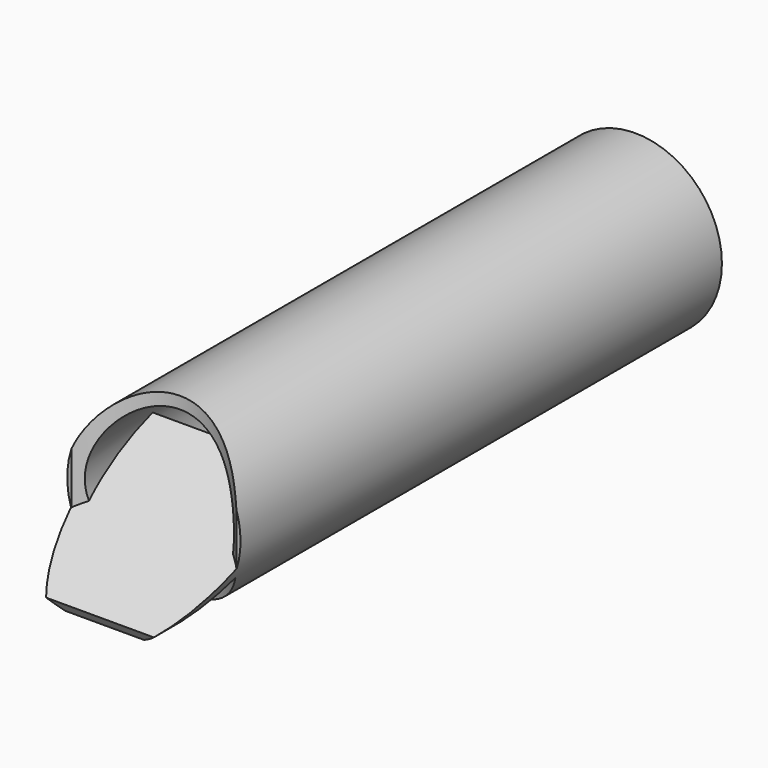
from build123d import *

# Parameters (mm, degrees)
F0_R     = 3.6
F0_R_2   = 3.1
F1_DEPTH = 12.5
F2_R     = 5
F3_DEPTH = 12.5
F5_DEPTH = 4
F6_R     = 5.6839494551
F6_R_2   = 3.6
F7_DEPTH = 25


# Not quite as in the source:
# - a feature names something its author has since deleted; it is built from what else it names


with BuildPart() as f1:
    # F0 (on Front) → F1 (new body, symmetric)
    with BuildSketch(Plane.XZ):
        Circle(F0_R)
        Circle(F0_R_2, mode=Mode.SUBTRACT)
    extrude(amount=F1_DEPTH, both=True)

    # F2 (on Top) → F3 (cut, symmetric)
    with BuildSketch(Plane.XY):
        with Locations((0, -16.1383841203)):
            Circle(F2_R)
    extrude(amount=F3_DEPTH, both=True, mode=Mode.SUBTRACT)

    # F4 (on Right) → F5 (join, symmetric)
    with BuildSketch(Plane.YZ):
        Polygon((-15.2992176846, -2.8184308636), (-15.0516938496, -3.2091679669), (-8.7361828689, 0.7915769966), (-8.9837067039, 1.1823140999), align=None)
    extrude(amount=F5_DEPTH, both=True)

    # F6 (on Front) → F7 (cut, symmetric)
    with BuildSketch(Plane.XZ):
        Circle(F6_R)
        Circle(F6_R_2, mode=Mode.SUBTRACT)
    extrude(amount=F7_DEPTH, both=True, mode=Mode.SUBTRACT)


solid = f1.part
